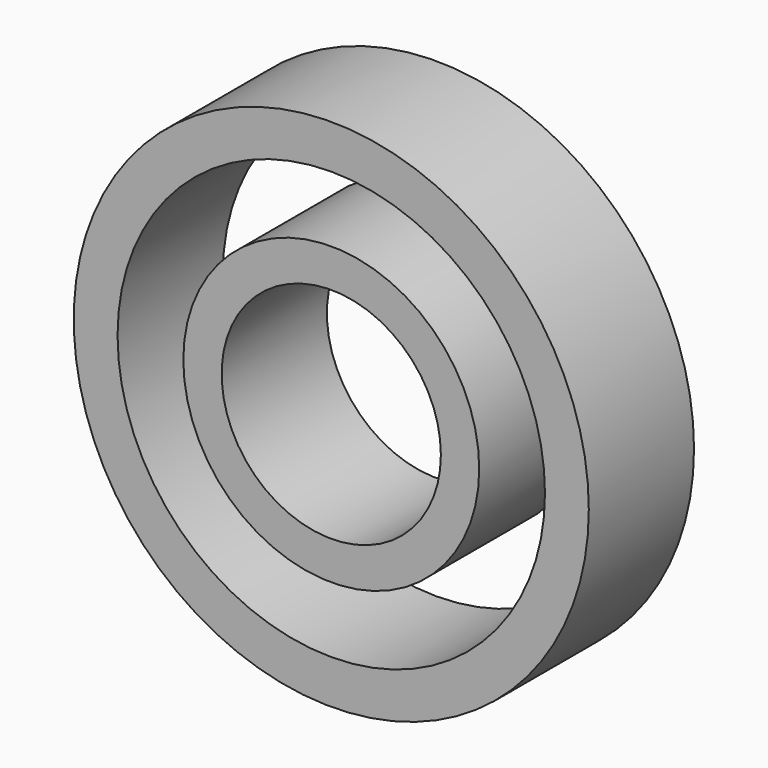
from build123d import *

# Parameters (mm, degrees)
F0_R     = 13.5
F0_R_2   = 10
F1_DEPTH = 12
F2_R     = 23.5
F2_R_2   = 19.5
F3_DEPTH = 12


# Not quite as in the source:
# - a feature of the source that left no trace in its solid (it failed there, or was rolled back) is left out
# - the program builds the solid bodies; features that only make, move or delete a surface that nothing else refers to are left out


with BuildPart() as f1:
    # F0 (on Front) → F1 (new body)
    with BuildSketch(Plane.XZ):
        Circle(F0_R)
        Circle(F0_R_2, mode=Mode.SUBTRACT)
    extrude(amount=F1_DEPTH)


with BuildPart() as f3:
    # F2 (on Front) → F3 (new body)
    with BuildSketch(Plane.XZ):
        Circle(F2_R)
        Circle(F2_R_2, mode=Mode.SUBTRACT)
    extrude(amount=F3_DEPTH)


solid = Compound([f1.part, f3.part])
